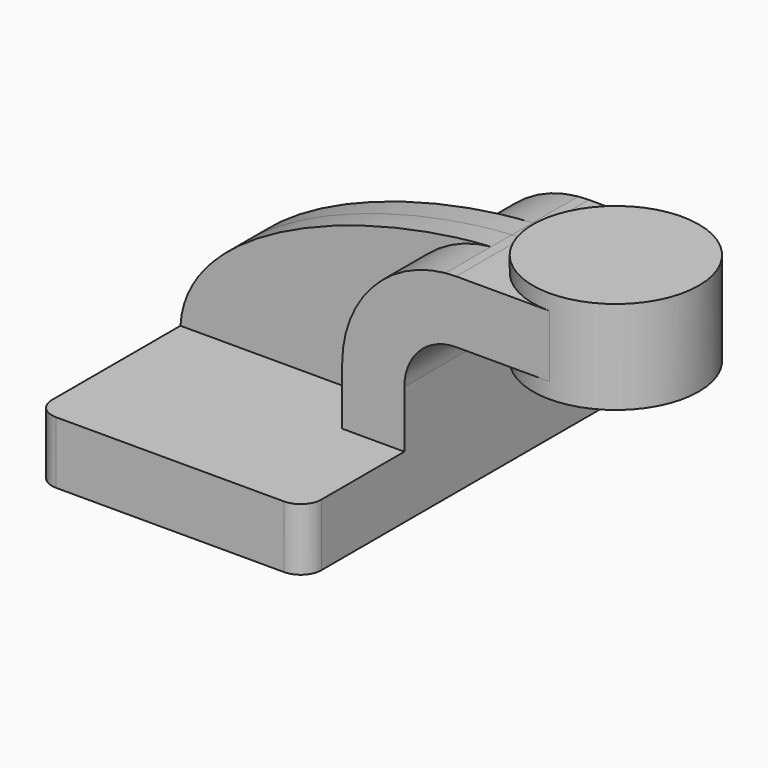
from build123d import *

# Parameters (mm, degrees)
F1_DEPTH = 63.5
F0_W     = 25.4
F0_H     = 19.05
F2_DEPTH = 25.4
F3_DEPTH = 7.9375
F5_R     = 6.35


# Not quite as in the source:
# - a feature of the source that left no trace in its solid (it failed there, or was rolled back) is left out


with BuildPart() as f1:
    # F0 (on Front) → F1 (new body, symmetric)
    with BuildSketch(Plane.XZ):
        Polygon((22.225, 9.525), (-41.275, 9.525), (-41.275, -9.525), (41.275, -9.525), (41.275, 9.525), align=None)
    extrude(amount=F1_DEPTH, both=True)

    # F0 (on Front) → F2 (join, symmetric)
    with BuildSketch(Plane.XZ):
        with BuildLine():
            Line((22.225, 27.0002), (22.225, 9.525))
            Line((22.225, 9.525), (41.275, 9.525))
            Line((41.275, 9.525), (41.275, 27.0002))
            ThreePointArc((41.275, 27.0002), (45.9246798487, 38.2255201513), (57.15, 42.8752))
            Line((57.15, 42.8752), (60.325, 42.8752))
            Line((60.325, 42.8752), (60.325, 61.9252))
            Line((60.325, 61.9252), (57.15, 61.9252))
            add(Edge.make_bspline(
                [(53.8854342407, 61.7722898912), (54.9842067368, 61.8365871986), (56.0728453275, 61.8876096574), (57.15, 61.9252)],
                knots=[108.5245810491, 108.5245810491, 108.5245810491, 108.5245810491, 111.5045361635, 111.5045361635, 111.5045361635, 111.5045361635], degree=3))
            ThreePointArc((53.8854342407, 61.7722898912), (31.3258777096, 50.5133948686), (22.225, 27.0002))
        make_face()
        with Locations((73.025, 52.4002)):
            Rectangle(F0_W, F0_H)
    extrude(amount=F2_DEPTH, both=True)

    # F0 (on Front) → F3 (join, symmetric)
    with BuildSketch(Plane.XZ):
        with BuildLine():
            add(Edge.make_bspline(
                [(-41.275, 9.525), (-39.5856284224, 39.4828766469), (13.870125209, 59.4306981306), (53.8854342407, 61.7722898912)],
                knots=[0, 0, 0, 0, 108.5245810491, 108.5245810491, 108.5245810491, 108.5245810491], degree=3))
            Line((-41.275, 9.525), (22.225, 9.525))
            Line((22.225, 9.525), (22.225, 27.0002))
            ThreePointArc((22.225, 27.0002), (31.3258777096, 50.5133948686), (53.8854342407, 61.7722898912))
        make_face()
    extrude(amount=F3_DEPTH, both=True)

    # F0 (on Front) → F4 (revolve)
    with BuildSketch(Plane.XZ):
        Polygon((85.725, 66.675), (85.725, 61.9252), (85.725, 42.8752), (85.725, 38.1), (111.125, 38.1), (111.125, 66.675), align=None)
    revolve(axis=Axis((85.725, 0, 52.3875), (0, 0, 1)))

    # F5
    f5_edges = [f1.edges().sort_by_distance(p)[0] for p in [
        (-41.275, -63.5, 0),
        (41.275, -63.5, 0),
        (-41.275, 63.5, 0),
        (41.275, 63.5, 0),
    ]]
    fillet(f5_edges, radius=F5_R)


solid = f1.part
